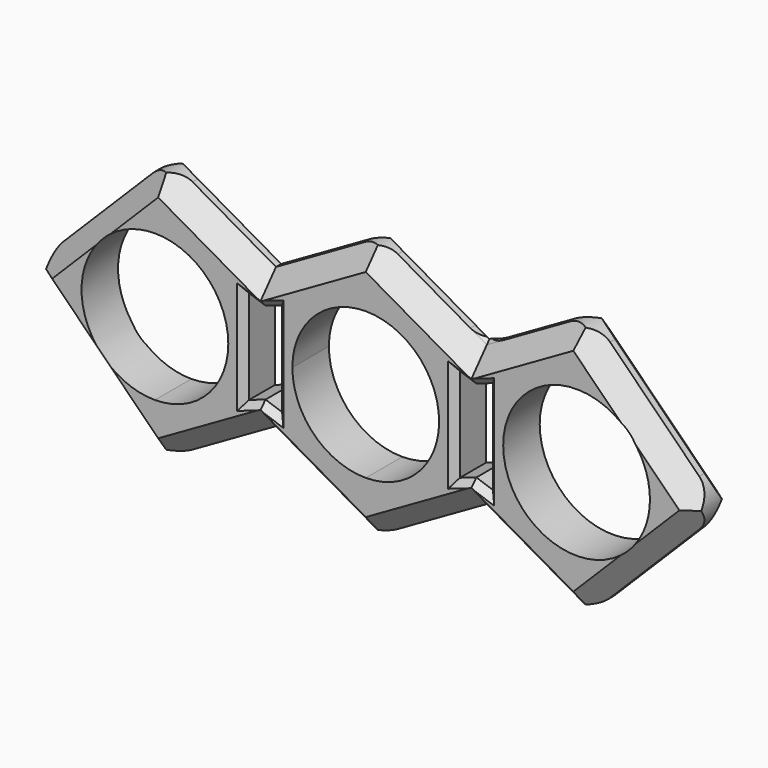
from build123d import *

# Parameters (mm, degrees)
F1_DEPTH      = 7
F3_DEPTH      = 127
F4_T1_DEPTH   = 43.7143691753
F4_T3_DEPTH   = 43.7143691753
F4_T5_DEPTH   = 43.7143691753
F4_T7_DEPTH   = 43.7143691753
F4_T12_DEPTH  = 34.0552517656
F4_T17_DEPTH  = 34.0552517656
F4_T22_DEPTH  = 34.0552517656
F4_T27_DEPTH  = 34.0552517656
F4_T32_DEPTH  = 34.0552517656
F4_T37_DEPTH  = 34.0552517656
F4_T42_DEPTH  = 34.0552517656
F4_T47_DEPTH  = 34.0552517656
F4_T52_DEPTH  = 34.0552517656
F4_T57_DEPTH  = 34.0552517656
F4_T62_DEPTH  = 34.0552517656
F4_T67_DEPTH  = 34.0552517656
F4_T72_DEPTH  = 34.0552517656
F4_T77_DEPTH  = 34.0552517656
F4_T82_DEPTH  = 34.0552517656
F4_T87_DEPTH  = 34.0552517656
F4_T93_DEPTH  = 34.0552517656
F4_T97_DEPTH  = 34.0552517656
F4_T104_DEPTH = 34.0552517656
F4_T108_DEPTH = 34.0552517656
F4_T115_DEPTH = 34.0552517656
F4_T119_DEPTH = 34.0552517656
F4_T126_DEPTH = 34.0552517656
F4_T130_DEPTH = 34.0552517656
F4_T137_DEPTH = 34.0552517656
F4_T141_DEPTH = 34.0552517656
F4_T148_DEPTH = 34.0552517656
F4_T152_DEPTH = 34.0552517656
F4_T159_DEPTH = 34.0552517656
F4_T163_DEPTH = 34.0552517656
F4_T170_DEPTH = 34.0552517656
F4_T174_DEPTH = 34.0552517656
F5_T4_DEPTH   = 15.5437371567
F5_T10_DEPTH  = 15.5437371567
F5_T16_DEPTH  = 15.5437371567
F5_T19_DEPTH  = 26.4
F5_T21_DEPTH  = 20.4179884798
F5_T23_DEPTH  = 15.5437371567
F6_T4_DEPTH   = 19.5677673114
F6_T10_DEPTH  = 19.5677673114
F6_T16_DEPTH  = 19.5677673114
F6_T22_DEPTH  = 19.5677673114
F6_T28_DEPTH  = 19.5677673114
F6_T34_DEPTH  = 19.5677673114
F6_T40_DEPTH  = 19.5677673114
F6_T46_DEPTH  = 19.5677673114
F6_T52_DEPTH  = 7.8272082618
F6_T57_DEPTH  = 7.8272082618
F6_T62_DEPTH  = 7.8272082618
F6_T67_DEPTH  = 7.8272082618
F6_T72_DEPTH  = 7.8272082618
F6_T77_DEPTH  = 7.8272082618
F6_T82_DEPTH  = 7.8272082618
F6_T87_DEPTH  = 7.8272082618
F6_T92_DEPTH  = 7.8272082618
F6_T97_DEPTH  = 7.8272082618
F6_T102_DEPTH = 7.8272082618
F6_T107_DEPTH = 7.8272082618
F6_T112_DEPTH = 7.8272082618
F6_T117_DEPTH = 7.8272082618
F6_T122_DEPTH = 7.8272082618
F6_T127_DEPTH = 7.8272082618
F6_T133_DEPTH = 7.8272082618
F6_T137_DEPTH = 19.5677673114
F6_T144_DEPTH = 7.8272082618
F6_T148_DEPTH = 19.5677673114
F6_T155_DEPTH = 19.5677673114
F6_T159_DEPTH = 7.8272082618
F6_T166_DEPTH = 7.8272082618
F6_T170_DEPTH = 19.5677673114
F6_T177_DEPTH = 19.5677673114
F6_T181_DEPTH = 7.8272082618
F6_T188_DEPTH = 7.8272082618
F6_T192_DEPTH = 19.5677673114
F6_T199_DEPTH = 7.8272082618
F6_T203_DEPTH = 19.5677673114
F6_T210_DEPTH = 7.8272082618
F6_T214_DEPTH = 19.5677673114
F6_T221_DEPTH = 7.8272082618
F6_T225_DEPTH = 19.5677673114
F6_T232_DEPTH = 7.8272082618
F6_T236_DEPTH = 19.5677673114
F6_T243_DEPTH = 19.5677673114
F6_T247_DEPTH = 7.8272082618
F6_T254_DEPTH = 7.8272082618
F6_T258_DEPTH = 19.5677673114
F6_T265_DEPTH = 19.5677673114
F6_T269_DEPTH = 7.8272082618
F6_T276_DEPTH = 7.8272082618
F6_T280_DEPTH = 19.5677673114
F6_T287_DEPTH = 7.8272082618
F6_T291_DEPTH = 19.5677673114
F6_T298_DEPTH = 7.8272082618
F6_T302_DEPTH = 19.5677673114


# Not quite as in the source:
# - a fillet or chamfer that OpenCascade refuses, or shapes differently, is made with other operations: its cross-section is extruded or revolved along the edge and cut away or added


with BuildPart() as f1:
    # F0 (on Front) → F1 (new body)
    with BuildSketch(Plane.XZ):
        with BuildLine():
            Line((16.1630827934, 10.7452115044), (16.1630827934, 0))
            Line((16.1630827934, 0), (21.0761655867, 0))
            ThreePointArc((21.0761655867, 0), (32.3261655867, 11.25), (43.5761655867, 0))
            Line((43.5761655867, 0), (52.3261655867, 0))
            Line((52.3261655867, 0), (32.3261655867, 20))
            Line((32.3261655867, 20), (16.1630827934, 10.7452115044))
        make_face()
        with BuildLine():
            Line((21.0761655867, 0), (16.1630827934, 0))
            Line((16.1630827934, 0), (16.1630827934, -10.7452115044))
            Line((16.1630827934, -10.7452115044), (32.3261655867, -20))
            Line((32.3261655867, -20), (52.3261655867, 0))
            Line((52.3261655867, 0), (43.5761655867, 0))
            ThreePointArc((43.5761655867, 0), (32.3261655867, -11.25), (21.0761655867, 0))
        make_face()
        with BuildLine():
            Line((16.1630827934, 0), (11.25, 0))
            ThreePointArc((11.25, 0), (7.9549512883, -7.9549512883), (0, -11.25))
            Line((0, -11.25), (0, -20))
            Line((0, -20), (16.1630827934, -10.7452115044))
            Line((16.1630827934, -10.7452115044), (16.1630827934, 0))
        make_face()
        with BuildLine():
            ThreePointArc((0, 11.25), (7.9549512883, 7.9549512883), (11.25, 0))
            Line((11.25, 0), (16.1630827934, 0))
            Line((16.1630827934, 0), (16.1630827934, 10.7452115044))
            Line((16.1630827934, 10.7452115044), (0, 20))
            Line((0, 20), (0, 11.25))
        make_face()
        with BuildLine():
            ThreePointArc((-11.25, 0), (-7.9549512883, 7.9549512883), (0, 11.25))
            Line((0, 11.25), (0, 20))
            Line((0, 20), (-16.1630827934, 10.7452115044))
            Line((-16.1630827934, 10.7452115044), (-16.1630827934, 0))
            Line((-16.1630827934, 0), (-11.25, 0))
        make_face()
        with BuildLine():
            Line((0, -20), (0, -11.25))
            ThreePointArc((0, -11.25), (-7.9549512883, -7.9549512883), (-11.25, 0))
            Line((-11.25, 0), (-16.1630827934, 0))
            Line((-16.1630827934, 0), (-16.1630827934, -10.7452115044))
            Line((-16.1630827934, -10.7452115044), (0, -20))
        make_face()
        with BuildLine():
            Line((-16.1630827934, -10.7452115044), (-16.1630827934, 0))
            Line((-16.1630827934, 0), (-21.0761655867, 0))
            ThreePointArc((-21.0761655867, 0), (-24.3712142984, -7.9549512883), (-32.3261655867, -11.25))
            Line((-32.3261655867, -11.25), (-32.3261655867, -20))
            Line((-32.3261655867, -20), (-16.1630827934, -10.7452115044))
        make_face()
        with BuildLine():
            Line((-52.3261655867, 0), (-32.3261655867, -20))
            Line((-32.3261655867, -20), (-32.3261655867, -11.25))
            ThreePointArc((-32.3261655867, -11.25), (-40.2811168751, -7.9549512883), (-43.5761655867, 0))
            Line((-43.5761655867, 0), (-52.3261655867, 0))
        make_face()
        with BuildLine():
            Line((-32.3261655867, 11.25), (-32.3261655867, 20))
            Line((-32.3261655867, 20), (-52.3261655867, 0))
            Line((-52.3261655867, 0), (-43.5761655867, 0))
            ThreePointArc((-43.5761655867, 0), (-40.2811168751, 7.9549512883), (-32.3261655867, 11.25))
        make_face()
        with BuildLine():
            Line((-21.0761655867, 0), (-16.1630827934, 0))
            Line((-16.1630827934, 0), (-16.1630827934, 10.7452115044))
            Line((-16.1630827934, 10.7452115044), (-32.3261655867, 20))
            Line((-32.3261655867, 20), (-32.3261655867, 11.25))
            ThreePointArc((-32.3261655867, 11.25), (-24.3712142984, 7.9549512883), (-21.0761655867, 0))
        make_face()
    extrude(amount=F1_DEPTH)

    # F2 (on face) → F3 (cut)
    with BuildSketch(Plane.XZ.offset(7)):
        Polygon((-16.1630827934, 6.3396666324), (-16.1630827934, -6.3396666324), (-13.6250335872, -7.2122006677), (-13.6250335872, 7.2122006677), align=None)
        Polygon((-18.7011319995, -7.2122006677), (-16.1630827934, -6.3396666324), (-16.1630827934, 6.3396666324), (-18.7011319995, 7.2122006677), align=None)
        Polygon((13.6250335872, -7.2122006677), (16.1630827934, -6.3396666324), (16.1630827934, 6.3396666324), (13.6250335872, 7.2122006677), align=None)
        Polygon((16.1630827934, 6.3396666324), (16.1630827934, -6.3396666324), (18.7011319995, -7.2122006677), (18.7011319995, 7.2122006677), align=None)
    extrude(amount=-F3_DEPTH, mode=Mode.SUBTRACT)

    # F4: chamfer of 3 on 24 edges, made by hand

    # F4_s2 → F4_t1 (cut)
    with BuildSketch(Plane(origin=(31.6184462329, 0, -31.6184462329), x_dir=(0, 1, 0), z_dir=(-0.7071067812, 0, 0.7071067812))):
        Polygon((-7, -34.0001865199), (-4, -37.0001865199), (-7, -37.0001865199), align=None)
        Polygon((0, -34.0001865199), (-3, -37.0001865199), (0, -37.0001865199), align=None)
    extrude(amount=F4_T1_DEPTH, mode=Mode.SUBTRACT)

    # F4_s4 → F4_t3 (cut)
    with BuildSketch(Plane(origin=(-0.7077193538, 0, -0.7077193538), x_dir=(0, 1, 0), z_dir=(-0.7071067812, 0, -0.7071067812))):
        Polygon((-7, -34.0001865199), (-4, -37.0001865199), (-7, -37.0001865199), align=None)
        Polygon((0, -34.0001865199), (-3, -37.0001865199), (0, -37.0001865199), align=None)
    extrude(amount=F4_T3_DEPTH, mode=Mode.SUBTRACT)

    # F4_s6 → F4_t5 (cut)
    with BuildSketch(Plane(origin=(-31.6184462329, 0, 31.6184462329), x_dir=(0, 1, 0), z_dir=(0.7071067812, 0, -0.7071067812))):
        Polygon((-7, -34.0001865199), (-4, -37.0001865199), (-7, -37.0001865199), align=None)
        Polygon((0, -34.0001865199), (-3, -37.0001865199), (0, -37.0001865199), align=None)
    extrude(amount=F4_T5_DEPTH, mode=Mode.SUBTRACT)

    # F4_s8 → F4_t7 (cut)
    with BuildSketch(Plane(origin=(0.7077193538, 0, 0.7077193538), x_dir=(0, 1, 0), z_dir=(0.7071067812, 0, 0.7071067812))):
        Polygon((0, -34.0001865199), (-3, -37.0001865199), (0, -37.0001865199), align=None)
        Polygon((-7, -34.0001865199), (-4, -37.0001865199), (-7, -37.0001865199), align=None)
    extrude(amount=F4_T7_DEPTH, mode=Mode.SUBTRACT)


with BuildPart() as f4_tool10:
    # F4_s11 → F4_t12 (new body)
    with BuildSketch(Plane(origin=(-10.1105795702, 0, 5.7891973138), x_dir=(0, 1, 0), z_dir=(-0.8678093579, 0, 0.4968972915))):
        Polygon((-7, 1.7065969657), (-4, -1.2934030343), (-7, -1.2934030343), align=None)
    extrude(amount=F4_T12_DEPTH)

    split(bisect_by=Plane(origin=(-8.6242423897, 0, 15.0618616342), x_dir=(0, 1, 0), z_dir=(-0.4968972915, 0, 0.8678093579)), keep=Keep.TOP)


with BuildPart() as f1_1:
    add(f1.part)

    # F4_t9: cut F4_tool10
    add(f4_tool10.part, mode=Mode.SUBTRACT)


with BuildPart() as f4_tool15:
    # F4_s16 → F4_t17 (new body)
    with BuildSketch(Plane(origin=(15.3194340774, 0, 8.7717252997), x_dir=(0, 1, 0), z_dir=(-0.8678093579, 0, -0.4968972915))):
        Polygon((-7, -14.3561871586), (-4, -17.3561871586), (-7, -17.3561871586), align=None)
    extrude(amount=F4_T17_DEPTH)

    split(bisect_by=Plane(origin=(0.6426884646, 0, 1.1224272567), x_dir=(0, 1, 0), z_dir=(0.4968972915, 0, 0.8678093579)), keep=Keep.TOP)


with BuildPart() as f1_2:
    add(f1_1.part)

    # F4_t14: cut F4_tool15
    add(f4_tool15.part, mode=Mode.SUBTRACT)


with BuildPart() as f4_tool20:
    # F4_s21 → F4_t22 (new body)
    with BuildSketch(Plane(origin=(14.2340320914, 0, -8.1502370637), x_dir=(0, 1, 0), z_dir=(-0.8678093579, 0, 0.4968972915))):
        Polygon((-7, -14.3561871586), (-4, -17.3561871586), (-7, -17.3561871586), align=None)
    extrude(amount=F4_T22_DEPTH)

    split(bisect_by=Plane(origin=(-0.6426884646, 0, 1.1224272567), x_dir=(0, 1, 0), z_dir=(-0.4968972915, 0, 0.8678093579)), keep=Keep.TOP)


with BuildPart() as f1_3:
    add(f1_2.part)

    # F4_t19: cut F4_tool20
    add(f4_tool20.part, mode=Mode.SUBTRACT)


with BuildPart() as f4_tool25:
    # F4_s26 → F4_t27 (new body)
    with BuildSketch(Plane(origin=(39.664045739, 0, 22.7111596771), x_dir=(0, 1, 0), z_dir=(-0.8678093579, 0, -0.4968972915))):
        Polygon((-7, 1.7065969657), (-4, -1.2934030343), (-7, -1.2934030343), align=None)
    extrude(amount=F4_T27_DEPTH)

    split(bisect_by=Plane(origin=(8.6242423897, 0, 15.0618616342), x_dir=(0, 1, 0), z_dir=(0.4968972915, 0, 0.8678093579)), keep=Keep.TOP)


with BuildPart() as f1_4:
    add(f1_3.part)

    # F4_t24: cut F4_tool25
    add(f4_tool25.part, mode=Mode.SUBTRACT)


with BuildPart() as f4_tool30:
    # F4_s31 → F4_t32 (new body)
    with BuildSketch(Plane(origin=(39.664045739, 0, 22.7111596771), x_dir=(0, 1, 0), z_dir=(-0.8678093579, 0, -0.4968972915))):
        Polygon((0, 1.7065969657), (-3, -1.2934030343), (0, -1.2934030343), align=None)
    extrude(amount=F4_T32_DEPTH)

    split(bisect_by=Plane(origin=(8.6242423897, 0, 15.0618616342), x_dir=(0, 1, 0), z_dir=(0.4968972915, 0, 0.8678093579)), keep=Keep.TOP)


with BuildPart() as f1_5:
    add(f1_4.part)

    # F4_t29: cut F4_tool30
    add(f4_tool30.part, mode=Mode.SUBTRACT)


with BuildPart() as f4_tool35:
    # F4_s36 → F4_t37 (new body)
    with BuildSketch(Plane(origin=(14.2340320914, 0, -8.1502370637), x_dir=(0, 1, 0), z_dir=(-0.8678093579, 0, 0.4968972915))):
        Polygon((0, -14.3561871586), (-3, -17.3561871586), (0, -17.3561871586), align=None)
    extrude(amount=F4_T37_DEPTH)

    split(bisect_by=Plane(origin=(-0.6426884646, 0, 1.1224272567), x_dir=(0, 1, 0), z_dir=(-0.4968972915, 0, 0.8678093579)), keep=Keep.TOP)


with BuildPart() as f1_6:
    add(f1_5.part)

    # F4_t34: cut F4_tool35
    add(f4_tool35.part, mode=Mode.SUBTRACT)


with BuildPart() as f4_tool40:
    # F4_s41 → F4_t42 (new body)
    with BuildSketch(Plane(origin=(15.3194340774, 0, 8.7717252997), x_dir=(0, 1, 0), z_dir=(-0.8678093579, 0, -0.4968972915))):
        Polygon((0, -14.3561871586), (-3, -17.3561871586), (0, -17.3561871586), align=None)
    extrude(amount=F4_T42_DEPTH)

    split(bisect_by=Plane(origin=(0.6426884646, 0, 1.1224272567), x_dir=(0, 1, 0), z_dir=(0.4968972915, 0, 0.8678093579)), keep=Keep.TOP)


with BuildPart() as f1_7:
    add(f1_6.part)

    # F4_t39: cut F4_tool40
    add(f4_tool40.part, mode=Mode.SUBTRACT)


with BuildPart() as f4_tool45:
    # F4_s46 → F4_t47 (new body)
    with BuildSketch(Plane(origin=(-10.1105795702, 0, 5.7891973138), x_dir=(0, 1, 0), z_dir=(-0.8678093579, 0, 0.4968972915))):
        Polygon((0, 1.7065969657), (-3, -1.2934030343), (0, -1.2934030343), align=None)
    extrude(amount=F4_T47_DEPTH)

    split(bisect_by=Plane(origin=(-8.6242423897, 0, 15.0618616342), x_dir=(0, 1, 0), z_dir=(-0.4968972915, 0, 0.8678093579)), keep=Keep.TOP)


with BuildPart() as f1_8:
    add(f1_7.part)

    # F4_t44: cut F4_tool45
    add(f4_tool45.part, mode=Mode.SUBTRACT)


with BuildPart() as f4_tool50:
    # F4_s51 → F4_t52 (new body)
    with BuildSketch(Plane(origin=(-39.664045739, 0, -22.7111596771), x_dir=(0, 1, 0), z_dir=(0.8678093579, 0, 0.4968972915))):
        Polygon((0, 1.7065969657), (-3, -1.2934030343), (0, -1.2934030343), align=None)
    extrude(amount=F4_T52_DEPTH)

    split(bisect_by=Plane(origin=(-8.6242423897, 0, -15.0618616342), x_dir=(0, 1, 0), z_dir=(-0.4968972915, 0, -0.8678093579)), keep=Keep.TOP)


with BuildPart() as f1_9:
    add(f1_8.part)

    # F4_t49: cut F4_tool50
    add(f4_tool50.part, mode=Mode.SUBTRACT)


with BuildPart() as f4_tool55:
    # F4_s56 → F4_t57 (new body)
    with BuildSketch(Plane(origin=(-39.664045739, 0, -22.7111596771), x_dir=(0, 1, 0), z_dir=(0.8678093579, 0, 0.4968972915))):
        Polygon((-7, 1.7065969657), (-4, -1.2934030343), (-7, -1.2934030343), align=None)
    extrude(amount=F4_T57_DEPTH)

    split(bisect_by=Plane(origin=(-8.6242423897, 0, -15.0618616342), x_dir=(0, 1, 0), z_dir=(-0.4968972915, 0, -0.8678093579)), keep=Keep.TOP)


with BuildPart() as f1_10:
    add(f1_9.part)

    # F4_t54: cut F4_tool55
    add(f4_tool55.part, mode=Mode.SUBTRACT)


with BuildPart() as f4_tool60:
    # F4_s61 → F4_t62 (new body)
    with BuildSketch(Plane(origin=(-14.2340320914, 0, 8.1502370637), x_dir=(0, 1, 0), z_dir=(0.8678093579, 0, -0.4968972915))):
        Polygon((-4, -17.3561871586), (-7, -14.3561871586), (-7, -17.3561871586), align=None)
    extrude(amount=F4_T62_DEPTH)

    split(bisect_by=Plane(origin=(0.6426884646, 0, -1.1224272567), x_dir=(0, 1, 0), z_dir=(0.4968972915, 0, -0.8678093579)), keep=Keep.TOP)


with BuildPart() as f1_11:
    add(f1_10.part)

    # F4_t59: cut F4_tool60
    add(f4_tool60.part, mode=Mode.SUBTRACT)


with BuildPart() as f4_tool65:
    # F4_s66 → F4_t67 (new body)
    with BuildSketch(Plane(origin=(-14.2340320914, 0, 8.1502370637), x_dir=(0, 1, 0), z_dir=(0.8678093579, 0, -0.4968972915))):
        Polygon((-3, -17.3561871586), (0, -14.3561871586), (0, -17.3561871586), align=None)
    extrude(amount=F4_T67_DEPTH)

    split(bisect_by=Plane(origin=(0.6426884646, 0, -1.1224272567), x_dir=(0, 1, 0), z_dir=(0.4968972915, 0, -0.8678093579)), keep=Keep.TOP)


with BuildPart() as f1_12:
    add(f1_11.part)

    # F4_t64: cut F4_tool65
    add(f4_tool65.part, mode=Mode.SUBTRACT)


with BuildPart() as f4_tool70:
    # F4_s71 → F4_t72 (new body)
    with BuildSketch(Plane(origin=(-15.3194340774, 0, -8.7717252997), x_dir=(0, 1, 0), z_dir=(0.8678093579, 0, 0.4968972915))):
        Polygon((-3, -17.3561871586), (0, -14.3561871586), (0, -17.3561871586), align=None)
    extrude(amount=F4_T72_DEPTH)

    split(bisect_by=Plane(origin=(-0.6426884646, 0, -1.1224272567), x_dir=(0, 1, 0), z_dir=(-0.4968972915, 0, -0.8678093579)), keep=Keep.TOP)


with BuildPart() as f1_13:
    add(f1_12.part)

    # F4_t69: cut F4_tool70
    add(f4_tool70.part, mode=Mode.SUBTRACT)


with BuildPart() as f4_tool75:
    # F4_s76 → F4_t77 (new body)
    with BuildSketch(Plane(origin=(-15.3194340774, 0, -8.7717252997), x_dir=(0, 1, 0), z_dir=(0.8678093579, 0, 0.4968972915))):
        Polygon((-4, -17.3561871586), (-7, -14.3561871586), (-7, -17.3561871586), align=None)
    extrude(amount=F4_T77_DEPTH)

    split(bisect_by=Plane(origin=(-0.6426884646, 0, -1.1224272567), x_dir=(0, 1, 0), z_dir=(-0.4968972915, 0, -0.8678093579)), keep=Keep.TOP)


with BuildPart() as f1_14:
    add(f1_13.part)

    # F4_t74: cut F4_tool75
    add(f4_tool75.part, mode=Mode.SUBTRACT)


with BuildPart() as f4_tool80:
    # F4_s81 → F4_t82 (new body)
    with BuildSketch(Plane(origin=(10.1105795702, 0, -5.7891973138), x_dir=(0, 1, 0), z_dir=(0.8678093579, 0, -0.4968972915))):
        Polygon((-3, -1.2934030343), (0, 1.7065969657), (0, -1.2934030343), align=None)
    extrude(amount=F4_T82_DEPTH)

    split(bisect_by=Plane(origin=(8.6242423897, 0, -15.0618616342), x_dir=(0, 1, 0), z_dir=(0.4968972915, 0, -0.8678093579)), keep=Keep.TOP)


with BuildPart() as f1_15:
    add(f1_14.part)

    # F4_t79: cut F4_tool80
    add(f4_tool80.part, mode=Mode.SUBTRACT)


with BuildPart() as f4_tool85:
    # F4_s86 → F4_t87 (new body)
    with BuildSketch(Plane(origin=(10.1105795702, 0, -5.7891973138), x_dir=(0, 1, 0), z_dir=(0.8678093579, 0, -0.4968972915))):
        Polygon((-4, -1.2934030343), (-7, 1.7065969657), (-7, -1.2934030343), align=None)
    extrude(amount=F4_T87_DEPTH)

    split(bisect_by=Plane(origin=(8.6242423897, 0, -15.0618616342), x_dir=(0, 1, 0), z_dir=(0.4968972915, 0, -0.8678093579)), keep=Keep.TOP)


with BuildPart() as f1_16:
    add(f1_15.part)

    # F4_t84: cut F4_tool85
    add(f4_tool85.part, mode=Mode.SUBTRACT)


with BuildPart() as f4_tool91:
    # F4_s92 → F4_t93 (new body)
    with BuildSketch(Plane(origin=(-10.1105795702, 0, 5.7891973138), x_dir=(0, 1, 0), z_dir=(-0.8678093579, 0, 0.4968972915))):
        Polygon((-7, 1.7065969657), (-4, -1.2934030343), (-7, -1.2934030343), align=None)
    extrude(amount=F4_T93_DEPTH)

    split(bisect_by=Plane(origin=(-8.6242423897, 0, 15.0618616342), x_dir=(0, 1, 0), z_dir=(0.4968972915, 0, -0.8678093579)), keep=Keep.TOP)


with BuildPart() as f4_tool95:
    # F4_s96 → F4_t97 (new body)
    with BuildSketch(Plane(origin=(15.3194340774, 0, 8.7717252997), x_dir=(0, 1, 0), z_dir=(-0.8678093579, 0, -0.4968972915))):
        Polygon((-7, -14.3561871586), (-4, -17.3561871586), (-7, -17.3561871586), align=None)
    extrude(amount=F4_T97_DEPTH)

    split(bisect_by=Plane(origin=(0.6426884646, 0, 1.1224272567), x_dir=(0, 1, 0), z_dir=(-0.4968972915, 0, -0.8678093579)), keep=Keep.TOP)


with BuildPart() as f4_tool91_1:
    add(f4_tool91.part)

    # F4_t99: intersect F4_tool95
    add(f4_tool95.part, mode=Mode.INTERSECT)


with BuildPart() as f1_17:
    add(f1_16.part)

    # F4_t89: cut F4_tool91
    add(f4_tool91_1.part, mode=Mode.SUBTRACT)


with BuildPart() as f4_tool102:
    # F4_s103 → F4_t104 (new body)
    with BuildSketch(Plane(origin=(39.664045739, 0, 22.7111596771), x_dir=(0, 1, 0), z_dir=(-0.8678093579, 0, -0.4968972915))):
        Polygon((-7, 1.7065969657), (-4, -1.2934030343), (-7, -1.2934030343), align=None)
    extrude(amount=F4_T104_DEPTH)

    split(bisect_by=Plane(origin=(8.6242423897, 0, 15.0618616342), x_dir=(0, 1, 0), z_dir=(-0.4968972915, 0, -0.8678093579)), keep=Keep.TOP)


with BuildPart() as f4_tool106:
    # F4_s107 → F4_t108 (new body)
    with BuildSketch(Plane(origin=(14.2340320914, 0, -8.1502370637), x_dir=(0, 1, 0), z_dir=(-0.8678093579, 0, 0.4968972915))):
        Polygon((-7, -14.3561871586), (-4, -17.3561871586), (-7, -17.3561871586), align=None)
    extrude(amount=F4_T108_DEPTH)

    split(bisect_by=Plane(origin=(-0.6426884646, 0, 1.1224272567), x_dir=(0, 1, 0), z_dir=(0.4968972915, 0, -0.8678093579)), keep=Keep.TOP)


with BuildPart() as f4_tool102_1:
    add(f4_tool102.part)

    # F4_t110: intersect F4_tool106
    add(f4_tool106.part, mode=Mode.INTERSECT)


with BuildPart() as f1_18:
    add(f1_17.part)

    # F4_t100: cut F4_tool102
    add(f4_tool102_1.part, mode=Mode.SUBTRACT)


with BuildPart() as f4_tool113:
    # F4_s114 → F4_t115 (new body)
    with BuildSketch(Plane(origin=(39.664045739, 0, 22.7111596771), x_dir=(0, 1, 0), z_dir=(-0.8678093579, 0, -0.4968972915))):
        Polygon((0, 1.7065969657), (-3, -1.2934030343), (0, -1.2934030343), align=None)
    extrude(amount=F4_T115_DEPTH)

    split(bisect_by=Plane(origin=(8.6242423897, 0, 15.0618616342), x_dir=(0, 1, 0), z_dir=(-0.4968972915, 0, -0.8678093579)), keep=Keep.TOP)


with BuildPart() as f4_tool117:
    # F4_s118 → F4_t119 (new body)
    with BuildSketch(Plane(origin=(14.2340320914, 0, -8.1502370637), x_dir=(0, 1, 0), z_dir=(-0.8678093579, 0, 0.4968972915))):
        Polygon((0, -14.3561871586), (-3, -17.3561871586), (0, -17.3561871586), align=None)
    extrude(amount=F4_T119_DEPTH)

    split(bisect_by=Plane(origin=(-0.6426884646, 0, 1.1224272567), x_dir=(0, 1, 0), z_dir=(0.4968972915, 0, -0.8678093579)), keep=Keep.TOP)


with BuildPart() as f4_tool113_1:
    add(f4_tool113.part)

    # F4_t121: intersect F4_tool117
    add(f4_tool117.part, mode=Mode.INTERSECT)


with BuildPart() as f1_19:
    add(f1_18.part)

    # F4_t111: cut F4_tool113
    add(f4_tool113_1.part, mode=Mode.SUBTRACT)


with BuildPart() as f4_tool124:
    # F4_s125 → F4_t126 (new body)
    with BuildSketch(Plane(origin=(-10.1105795702, 0, 5.7891973138), x_dir=(0, 1, 0), z_dir=(-0.8678093579, 0, 0.4968972915))):
        Polygon((0, 1.7065969657), (-3, -1.2934030343), (0, -1.2934030343), align=None)
    extrude(amount=F4_T126_DEPTH)

    split(bisect_by=Plane(origin=(-8.6242423897, 0, 15.0618616342), x_dir=(0, 1, 0), z_dir=(0.4968972915, 0, -0.8678093579)), keep=Keep.TOP)


with BuildPart() as f4_tool128:
    # F4_s129 → F4_t130 (new body)
    with BuildSketch(Plane(origin=(15.3194340774, 0, 8.7717252997), x_dir=(0, 1, 0), z_dir=(-0.8678093579, 0, -0.4968972915))):
        Polygon((0, -14.3561871586), (-3, -17.3561871586), (0, -17.3561871586), align=None)
    extrude(amount=F4_T130_DEPTH)

    split(bisect_by=Plane(origin=(0.6426884646, 0, 1.1224272567), x_dir=(0, 1, 0), z_dir=(-0.4968972915, 0, -0.8678093579)), keep=Keep.TOP)


with BuildPart() as f4_tool124_1:
    add(f4_tool124.part)

    # F4_t132: intersect F4_tool128
    add(f4_tool128.part, mode=Mode.INTERSECT)


with BuildPart() as f1_20:
    add(f1_19.part)

    # F4_t122: cut F4_tool124
    add(f4_tool124_1.part, mode=Mode.SUBTRACT)


with BuildPart() as f4_tool135:
    # F4_s136 → F4_t137 (new body)
    with BuildSketch(Plane(origin=(-14.2340320914, 0, 8.1502370637), x_dir=(0, 1, 0), z_dir=(0.8678093579, 0, -0.4968972915))):
        Polygon((-3, -17.3561871586), (0, -14.3561871586), (0, -17.3561871586), align=None)
    extrude(amount=F4_T137_DEPTH)

    split(bisect_by=Plane(origin=(0.6426884646, 0, -1.1224272567), x_dir=(0, 1, 0), z_dir=(-0.4968972915, 0, 0.8678093579)), keep=Keep.TOP)


with BuildPart() as f4_tool139:
    # F4_s140 → F4_t141 (new body)
    with BuildSketch(Plane(origin=(-39.664045739, 0, -22.7111596771), x_dir=(0, 1, 0), z_dir=(0.8678093579, 0, 0.4968972915))):
        Polygon((0, 1.7065969657), (-3, -1.2934030343), (0, -1.2934030343), align=None)
    extrude(amount=F4_T141_DEPTH)

    split(bisect_by=Plane(origin=(-8.6242423897, 0, -15.0618616342), x_dir=(0, 1, 0), z_dir=(0.4968972915, 0, 0.8678093579)), keep=Keep.TOP)


with BuildPart() as f4_tool135_1:
    add(f4_tool135.part)

    # F4_t143: intersect F4_tool139
    add(f4_tool139.part, mode=Mode.INTERSECT)


with BuildPart() as f1_21:
    add(f1_20.part)

    # F4_t133: cut F4_tool135
    add(f4_tool135_1.part, mode=Mode.SUBTRACT)


with BuildPart() as f4_tool146:
    # F4_s147 → F4_t148 (new body)
    with BuildSketch(Plane(origin=(-14.2340320914, 0, 8.1502370637), x_dir=(0, 1, 0), z_dir=(0.8678093579, 0, -0.4968972915))):
        Polygon((-4, -17.3561871586), (-7, -14.3561871586), (-7, -17.3561871586), align=None)
    extrude(amount=F4_T148_DEPTH)

    split(bisect_by=Plane(origin=(0.6426884646, 0, -1.1224272567), x_dir=(0, 1, 0), z_dir=(-0.4968972915, 0, 0.8678093579)), keep=Keep.TOP)


with BuildPart() as f4_tool150:
    # F4_s151 → F4_t152 (new body)
    with BuildSketch(Plane(origin=(-39.664045739, 0, -22.7111596771), x_dir=(0, 1, 0), z_dir=(0.8678093579, 0, 0.4968972915))):
        Polygon((-7, 1.7065969657), (-4, -1.2934030343), (-7, -1.2934030343), align=None)
    extrude(amount=F4_T152_DEPTH)

    split(bisect_by=Plane(origin=(-8.6242423897, 0, -15.0618616342), x_dir=(0, 1, 0), z_dir=(0.4968972915, 0, 0.8678093579)), keep=Keep.TOP)


with BuildPart() as f4_tool146_1:
    add(f4_tool146.part)

    # F4_t154: intersect F4_tool150
    add(f4_tool150.part, mode=Mode.INTERSECT)


with BuildPart() as f1_22:
    add(f1_21.part)

    # F4_t144: cut F4_tool146
    add(f4_tool146_1.part, mode=Mode.SUBTRACT)


with BuildPart() as f4_tool157:
    # F4_s158 → F4_t159 (new body)
    with BuildSketch(Plane(origin=(-15.3194340774, 0, -8.7717252997), x_dir=(0, 1, 0), z_dir=(0.8678093579, 0, 0.4968972915))):
        Polygon((-3, -17.3561871586), (0, -14.3561871586), (0, -17.3561871586), align=None)
    extrude(amount=F4_T159_DEPTH)

    split(bisect_by=Plane(origin=(-0.6426884646, 0, -1.1224272567), x_dir=(0, 1, 0), z_dir=(0.4968972915, 0, 0.8678093579)), keep=Keep.TOP)


with BuildPart() as f4_tool161:
    # F4_s162 → F4_t163 (new body)
    with BuildSketch(Plane(origin=(10.1105795702, 0, -5.7891973138), x_dir=(0, 1, 0), z_dir=(0.8678093579, 0, -0.4968972915))):
        Polygon((-3, -1.2934030343), (0, 1.7065969657), (0, -1.2934030343), align=None)
    extrude(amount=F4_T163_DEPTH)

    split(bisect_by=Plane(origin=(8.6242423897, 0, -15.0618616342), x_dir=(0, 1, 0), z_dir=(-0.4968972915, 0, 0.8678093579)), keep=Keep.TOP)


with BuildPart() as f4_tool157_1:
    add(f4_tool157.part)

    # F4_t165: intersect F4_tool161
    add(f4_tool161.part, mode=Mode.INTERSECT)


with BuildPart() as f1_23:
    add(f1_22.part)

    # F4_t155: cut F4_tool157
    add(f4_tool157_1.part, mode=Mode.SUBTRACT)


with BuildPart() as f4_tool168:
    # F4_s169 → F4_t170 (new body)
    with BuildSketch(Plane(origin=(-15.3194340774, 0, -8.7717252997), x_dir=(0, 1, 0), z_dir=(0.8678093579, 0, 0.4968972915))):
        Polygon((-4, -17.3561871586), (-7, -14.3561871586), (-7, -17.3561871586), align=None)
    extrude(amount=F4_T170_DEPTH)

    split(bisect_by=Plane(origin=(-0.6426884646, 0, -1.1224272567), x_dir=(0, 1, 0), z_dir=(0.4968972915, 0, 0.8678093579)), keep=Keep.TOP)


with BuildPart() as f4_tool172:
    # F4_s173 → F4_t174 (new body)
    with BuildSketch(Plane(origin=(10.1105795702, 0, -5.7891973138), x_dir=(0, 1, 0), z_dir=(0.8678093579, 0, -0.4968972915))):
        Polygon((-4, -1.2934030343), (-7, 1.7065969657), (-7, -1.2934030343), align=None)
    extrude(amount=F4_T174_DEPTH)

    split(bisect_by=Plane(origin=(8.6242423897, 0, -15.0618616342), x_dir=(0, 1, 0), z_dir=(-0.4968972915, 0, 0.8678093579)), keep=Keep.TOP)


with BuildPart() as f4_tool168_1:
    add(f4_tool168.part)

    # F4_t176: intersect F4_tool172
    add(f4_tool172.part, mode=Mode.INTERSECT)


with BuildPart() as f1_24:
    add(f1_23.part)

    # F4_t166: cut F4_tool168
    add(f4_tool168_1.part, mode=Mode.SUBTRACT)

    # F5: fillet of radius 5.08 on 9 edges, made by hand


with BuildPart() as f5_tool2:
    # F5_s3 → F5_t4 (new body)
    with BuildSketch(Plane.XZ.offset(-4.2718685783)):
        with BuildLine():
            ThreePointArc((18.6873210341, 12.1905602247), (16.1630827934, 11.5190317629), (13.6388445526, 12.1905602247))
            Line((13.6388445526, 12.1905602247), (16.1630827934, 10.7452115044))
            Line((16.1630827934, 10.7452115044), (18.6873210341, 12.1905602247))
        make_face()
    extrude(amount=F5_T4_DEPTH)

    split(bisect_by=Plane(origin=(-1.3151388153, -2.6467015172, 2.2968323442), x_dir=(-0.8955358635, 0.444989345, 0), z_dir=(0.3513594444, 0.7071067812, -0.6136338818)), keep=Keep.TOP)

    split(bisect_by=Plane(origin=(3.5667752576, 7.1780935793, 6.2292167802), x_dir=(0.8955358635, -0.444989345, 0), z_dir=(-0.3513594444, -0.7071067812, -0.6136338818)), keep=Keep.TOP)


with BuildPart() as f1_25:
    add(f1_24.part)

    # F5_t1: union F5_tool2
    add(f5_tool2.part)


with BuildPart() as f5_tool8:
    # F5_s9 → F5_t10 (new body)
    with BuildSketch(Plane.XZ.offset(-4.2718685783)):
        with BuildLine():
            ThreePointArc((18.6873210341, 12.1905602247), (16.1630827934, 11.5190317629), (13.6388445526, 12.1905602247))
            Line((13.6388445526, 12.1905602247), (16.1630827934, 10.7452115044))
            Line((16.1630827934, 10.7452115044), (18.6873210341, 12.1905602247))
        make_face()
    extrude(amount=F5_T10_DEPTH)

    split(bisect_by=Plane(origin=(5.3059157778, -10.6780935793, 9.266549533), x_dir=(-0.8955358635, -0.444989345, 0), z_dir=(-0.3513594444, 0.7071067812, -0.6136338818)), keep=Keep.TOP)

    split(bisect_by=Plane(origin=(3.5667752576, 7.1780935793, 6.2292167802), x_dir=(0.8955358635, -0.444989345, 0), z_dir=(-0.3513594444, -0.7071067812, -0.6136338818)), keep=Keep.TOP)


with BuildPart() as f1_26:
    add(f1_25.part)

    # F5_t7: union F5_tool8
    add(f5_tool8.part)


with BuildPart() as f5_tool14:
    # F5_s15 → F5_t16 (new body)
    with BuildSketch(Plane.XZ.offset(-4.2718685783)):
        with BuildLine():
            ThreePointArc((18.6873210341, 12.1905602247), (16.1630827934, 11.5190317629), (13.6388445526, 12.1905602247))
            Line((13.6388445526, 12.1905602247), (16.1630827934, 10.7452115044))
            Line((16.1630827934, 10.7452115044), (18.6873210341, 12.1905602247))
        make_face()
    extrude(amount=F5_T16_DEPTH)

    split(bisect_by=Plane(origin=(-1.3151388153, -2.6467015171, 2.2968323442), x_dir=(-0.8955358635, 0.444989345, 0), z_dir=(0.3513594444, 0.7071067812, -0.6136338818)), keep=Keep.TOP)

    split(bisect_by=Plane(origin=(0.424001705, -0.8532984829, -0.7405004085), x_dir=(0.8955358635, 0.444989345, 0), z_dir=(0.3513594444, -0.7071067812, -0.6136338818)), keep=Keep.TOP)


with BuildPart() as f1_27:
    add(f1_26.part)

    # F5_t13: union F5_tool14
    add(f5_tool14.part)

    # F5_s20 → F5_t19 (cut)
    with BuildSketch(Plane.XZ.offset(-9.7)):
        with BuildLine():
            ThreePointArc((-48.7340631383, -3.5921024484), (-50.2219606899, 0), (-48.7340631383, 3.5921024484))
            Line((-48.7340631383, 3.5921024484), (-52.3261655867, 0))
            Line((-52.3261655867, 0), (-48.7340631383, -3.5921024484))
        make_face()
        with BuildLine():
            ThreePointArc((48.7340631383, -3.5921024484), (50.2219606899, 0), (48.7340631383, 3.5921024484))
            Line((48.7340631383, 3.5921024484), (52.3261655867, 0))
            Line((52.3261655867, 0), (48.7340631383, -3.5921024484))
        make_face()
    extrude(amount=F5_T19_DEPTH, mode=Mode.SUBTRACT)

    # F5_s22 → F5_t21 (cut)
    with BuildSketch(Plane.XZ.offset(-6.7089942399)):
        with BuildLine():
            ThreePointArc((-28.9559431637, -18.0702508236), (-32.1522663055, -18.6971245452), (-35.0722838529, -17.2538817338))
            Line((-35.0722838529, -17.2538817338), (-32.3261655867, -20))
            Line((-32.3261655867, -20), (-28.9559431637, -18.0702508236))
        make_face()
        with BuildLine():
            ThreePointArc((35.0722838529, -17.2538817338), (32.1522663055, -18.6971245452), (28.9559431637, -18.0702508236))
            Line((28.9559431637, -18.0702508236), (32.3261655867, -20))
            Line((32.3261655867, -20), (35.0722838529, -17.2538817338))
        make_face()
        with BuildLine():
            ThreePointArc((35.0722838529, 17.2538817338), (32.1522663055, 18.6971245452), (28.9559431637, 18.0702508236))
            Line((28.9559431637, 18.0702508236), (32.3261655867, 20))
            Line((32.3261655867, 20), (35.0722838529, 17.2538817338))
        make_face()
        with BuildLine():
            ThreePointArc((-35.0722838529, 17.2538817338), (-32.1522663055, 18.6971245452), (-28.9559431637, 18.0702508236))
            Line((-28.9559431637, 18.0702508236), (-32.3261655867, 20))
            Line((-32.3261655867, 20), (-35.0722838529, 17.2538817338))
        make_face()
    extrude(amount=F5_T21_DEPTH, mode=Mode.SUBTRACT)

    # F5_s24 → F5_t23 (cut)
    with BuildSketch(Plane.XZ.offset(-4.2718685783)):
        with BuildLine():
            ThreePointArc((-2.5242382408, -18.5546512797), (0, -19.2261797415), (2.5242382408, -18.5546512797))
            Line((2.5242382408, -18.5546512797), (0, -20))
            Line((0, -20), (-2.5242382408, -18.5546512797))
        make_face()
        with BuildLine():
            ThreePointArc((-2.5242382408, 18.5546512797), (0, 19.2261797415), (2.5242382408, 18.5546512797))
            Line((2.5242382408, 18.5546512797), (0, 20))
            Line((0, 20), (-2.5242382408, 18.5546512797))
        make_face()
    extrude(amount=F5_T23_DEPTH, mode=Mode.SUBTRACT)

    # F6: chamfer of 1 on 24 edges, made by hand


with BuildPart() as f6_tool2:
    # F6_s3 → F6_t4 (new body)
    with BuildSketch(Plane.XY.offset(-9.7838836557)):
        Polygon((-12.6250335872, 0), (-13.6250335872, -1), (-13.6250335872, 0), align=None)
    extrude(amount=F6_T4_DEPTH)

    split(bisect_by=Plane(origin=(-3.6574458748, 0, -10.6388716353), x_dir=(0, 1, 0), z_dir=(0.3251063, 0, 0.9456774787)), keep=Keep.TOP)

    split(bisect_by=Plane(origin=(-3.6574458748, 0, 10.6388716353), x_dir=(0, 1, 0), z_dir=(0.3251063, 0, -0.9456774787)), keep=Keep.TOP)


with BuildPart() as f1_28:
    add(f1_27.part)

    # F6_t1: cut F6_tool2
    add(f6_tool2.part, mode=Mode.SUBTRACT)


with BuildPart() as f6_tool8:
    # F6_s9 → F6_t10 (new body)
    with BuildSketch(Plane.XY.offset(9.7838836557)):
        Polygon((-19.7011319995, 0), (-18.7011319995, -1), (-18.7011319995, 0), align=None)
    extrude(amount=-F6_T10_DEPTH)

    split(bisect_by=Plane(origin=(0.2407606934, 0, -0.7003308317), x_dir=(0, 1, 0), z_dir=(-0.3251063, 0, 0.9456774787)), keep=Keep.TOP)

    split(bisect_by=Plane(origin=(0.2407606934, 0, 0.7003308317), x_dir=(0, 1, 0), z_dir=(-0.3251063, 0, -0.9456774787)), keep=Keep.TOP)


with BuildPart() as f1_29:
    add(f1_28.part)

    # F6_t7: cut F6_tool8
    add(f6_tool8.part, mode=Mode.SUBTRACT)


with BuildPart() as f6_tool14:
    # F6_s15 → F6_t16 (new body)
    with BuildSketch(Plane.XY.offset(9.7838836557)):
        Polygon((-18.7011319995, -6), (-19.7011319995, -7), (-18.7011319995, -7), align=None)
    extrude(amount=-F6_T16_DEPTH)

    split(bisect_by=Plane(origin=(0.2407606934, 0, -0.7003308317), x_dir=(0, 1, 0), z_dir=(-0.3251063, 0, 0.9456774787)), keep=Keep.TOP)

    split(bisect_by=Plane(origin=(0.2407606934, 0, 0.7003308317), x_dir=(0, 1, 0), z_dir=(-0.3251063, 0, -0.9456774787)), keep=Keep.TOP)


with BuildPart() as f1_30:
    add(f1_29.part)

    # F6_t13: cut F6_tool14
    add(f6_tool14.part, mode=Mode.SUBTRACT)


with BuildPart() as f6_tool20:
    # F6_s21 → F6_t22 (new body)
    with BuildSketch(Plane.XY.offset(-9.7838836557)):
        Polygon((-13.6250335872, -6), (-12.6250335872, -7), (-13.6250335872, -7), align=None)
    extrude(amount=F6_T22_DEPTH)

    split(bisect_by=Plane(origin=(-3.6574458748, 0, -10.6388716353), x_dir=(0, 1, 0), z_dir=(0.3251063, 0, 0.9456774787)), keep=Keep.TOP)

    split(bisect_by=Plane(origin=(-3.6574458748, 0, 10.6388716353), x_dir=(0, 1, 0), z_dir=(0.3251063, 0, -0.9456774787)), keep=Keep.TOP)


with BuildPart() as f1_31:
    add(f1_30.part)

    # F6_t19: cut F6_tool20
    add(f6_tool20.part, mode=Mode.SUBTRACT)


with BuildPart() as f6_tool26:
    # F6_s27 → F6_t28 (new body)
    with BuildSketch(Plane.XY.offset(9.7838836557)):
        Polygon((13.6250335872, -6), (12.6250335872, -7), (13.6250335872, -7), align=None)
    extrude(amount=-F6_T28_DEPTH)

    split(bisect_by=Plane(origin=(3.6574458748, 0, 10.6388716353), x_dir=(0, 1, 0), z_dir=(-0.3251063, 0, -0.9456774787)), keep=Keep.TOP)

    split(bisect_by=Plane(origin=(3.6574458748, 0, -10.6388716353), x_dir=(0, 1, 0), z_dir=(-0.3251063, 0, 0.9456774787)), keep=Keep.TOP)


with BuildPart() as f1_32:
    add(f1_31.part)

    # F6_t25: cut F6_tool26
    add(f6_tool26.part, mode=Mode.SUBTRACT)


with BuildPart() as f6_tool32:
    # F6_s33 → F6_t34 (new body)
    with BuildSketch(Plane.XY.offset(-9.7838836557)):
        Polygon((18.7011319995, -6), (19.7011319995, -7), (18.7011319995, -7), align=None)
    extrude(amount=F6_T34_DEPTH)

    split(bisect_by=Plane(origin=(-0.2407606934, 0, 0.7003308317), x_dir=(0, 1, 0), z_dir=(0.3251063, 0, -0.9456774787)), keep=Keep.TOP)

    split(bisect_by=Plane(origin=(-0.2407606934, 0, -0.7003308317), x_dir=(0, 1, 0), z_dir=(0.3251063, 0, 0.9456774787)), keep=Keep.TOP)


with BuildPart() as f1_33:
    add(f1_32.part)

    # F6_t31: cut F6_tool32
    add(f6_tool32.part, mode=Mode.SUBTRACT)


with BuildPart() as f6_tool38:
    # F6_s39 → F6_t40 (new body)
    with BuildSketch(Plane.XY.offset(-9.7838836557)):
        Polygon((19.7011319995, 0), (18.7011319995, -1), (18.7011319995, 0), align=None)
    extrude(amount=F6_T40_DEPTH)

    split(bisect_by=Plane(origin=(-0.2407606934, 0, 0.7003308317), x_dir=(0, 1, 0), z_dir=(0.3251063, 0, -0.9456774787)), keep=Keep.TOP)

    split(bisect_by=Plane(origin=(-0.2407606934, 0, -0.7003308317), x_dir=(0, 1, 0), z_dir=(0.3251063, 0, 0.9456774787)), keep=Keep.TOP)


with BuildPart() as f1_34:
    add(f1_33.part)

    # F6_t37: cut F6_tool38
    add(f6_tool38.part, mode=Mode.SUBTRACT)


with BuildPart() as f6_tool44:
    # F6_s45 → F6_t46 (new body)
    with BuildSketch(Plane.XY.offset(9.7838836557)):
        Polygon((12.6250335872, 0), (13.6250335872, -1), (13.6250335872, 0), align=None)
    extrude(amount=-F6_T46_DEPTH)

    split(bisect_by=Plane(origin=(3.6574458748, 0, 10.6388716353), x_dir=(0, 1, 0), z_dir=(-0.3251063, 0, -0.9456774787)), keep=Keep.TOP)

    split(bisect_by=Plane(origin=(3.6574458748, 0, -10.6388716353), x_dir=(0, 1, 0), z_dir=(-0.3251063, 0, 0.9456774787)), keep=Keep.TOP)


with BuildPart() as f1_35:
    add(f1_34.part)

    # F6_t43: cut F6_tool44
    add(f6_tool44.part, mode=Mode.SUBTRACT)


with BuildPart() as f6_tool50:
    # F6_s51 → F6_t52 (new body)
    with BuildSketch(Plane(origin=(13.9718608027, 0, -4.8032654597), x_dir=(0, 1, 0), z_dir=(0.9456774787, 0, -0.3251063))):
        Polygon((0, -1.7405599134), (-1, -0.7405599134), (0, -0.7405599134), align=None)
    extrude(amount=F6_T52_DEPTH)

    split(bisect_by=Plane.YZ.offset(18.7011319995), keep=Keep.BOTTOM)


with BuildPart() as f1_36:
    add(f1_35.part)

    # F6_t49: cut F6_tool50
    add(f6_tool50.part, mode=Mode.SUBTRACT)


with BuildPart() as f6_tool55:
    # F6_s56 → F6_t57 (new body)
    with BuildSketch(Plane(origin=(7.5356050283, 0, 2.5906006266), x_dir=(0, 1, 0), z_dir=(0.9456774787, 0, 0.3251063))):
        Polygon((0, -12.25), (-1, -11.25), (0, -11.25), align=None)
    extrude(amount=F6_T57_DEPTH)

    split(bisect_by=Plane.YZ.offset(13.6250335872), keep=Keep.TOP)


with BuildPart() as f1_37:
    add(f1_36.part)

    # F6_t54: cut F6_tool55
    add(f6_tool55.part, mode=Mode.SUBTRACT)


with BuildPart() as f6_tool60:
    # F6_s61 → F6_t62 (new body)
    with BuildSketch(Plane(origin=(21.3738753769, 0, 7.347940177), x_dir=(0, 1, 0), z_dir=(-0.9456774787, 0, -0.3251063))):
        Polygon((0, -1.7405599134), (-1, -0.7405599134), (0, -0.7405599134), align=None)
    extrude(amount=F6_T62_DEPTH)

    split(bisect_by=Plane.YZ.offset(18.7011319995), keep=Keep.BOTTOM)


with BuildPart() as f1_38:
    add(f1_37.part)

    # F6_t59: cut F6_tool60
    add(f6_tool60.part, mode=Mode.SUBTRACT)


with BuildPart() as f6_tool65:
    # F6_s66 → F6_t67 (new body)
    with BuildSketch(Plane(origin=(14.9376196026, 0, -5.1352753439), x_dir=(0, 1, 0), z_dir=(-0.9456774787, 0, 0.3251063))):
        Polygon((0, -12.25), (-1, -11.25), (0, -11.25), align=None)
    extrude(amount=F6_T67_DEPTH)

    split(bisect_by=Plane.YZ.offset(13.6250335872), keep=Keep.TOP)


with BuildPart() as f1_39:
    add(f1_38.part)

    # F6_t64: cut F6_tool65
    add(f6_tool65.part, mode=Mode.SUBTRACT)


with BuildPart() as f6_tool70:
    # F6_s71 → F6_t72 (new body)
    with BuildSketch(Plane(origin=(14.9376196026, 0, -5.1352753439), x_dir=(0, 1, 0), z_dir=(-0.9456774787, 0, 0.3251063))):
        Polygon((-6, -11.25), (-7, -12.25), (-7, -11.25), align=None)
    extrude(amount=F6_T72_DEPTH)

    split(bisect_by=Plane.YZ.offset(13.6250335872), keep=Keep.TOP)


with BuildPart() as f1_40:
    add(f1_39.part)

    # F6_t69: cut F6_tool70
    add(f6_tool70.part, mode=Mode.SUBTRACT)


with BuildPart() as f6_tool75:
    # F6_s76 → F6_t77 (new body)
    with BuildSketch(Plane(origin=(21.3738753769, 0, 7.347940177), x_dir=(0, 1, 0), z_dir=(-0.9456774787, 0, -0.3251063))):
        Polygon((-6, -0.7405599134), (-7, -1.7405599134), (-7, -0.7405599134), align=None)
    extrude(amount=F6_T77_DEPTH)

    split(bisect_by=Plane.YZ.offset(18.7011319995), keep=Keep.BOTTOM)


with BuildPart() as f1_41:
    add(f1_40.part)

    # F6_t74: cut F6_tool75
    add(f6_tool75.part, mode=Mode.SUBTRACT)


with BuildPart() as f6_tool80:
    # F6_s81 → F6_t82 (new body)
    with BuildSketch(Plane(origin=(7.5356050283, 0, 2.5906006266), x_dir=(0, 1, 0), z_dir=(0.9456774787, 0, 0.3251063))):
        Polygon((-6, -11.25), (-7, -12.25), (-7, -11.25), align=None)
    extrude(amount=F6_T82_DEPTH)

    split(bisect_by=Plane.YZ.offset(13.6250335872), keep=Keep.TOP)


with BuildPart() as f1_42:
    add(f1_41.part)

    # F6_t79: cut F6_tool80
    add(f6_tool80.part, mode=Mode.SUBTRACT)


with BuildPart() as f6_tool85:
    # F6_s86 → F6_t87 (new body)
    with BuildSketch(Plane(origin=(13.9718608027, 0, -4.8032654597), x_dir=(0, 1, 0), z_dir=(0.9456774787, 0, -0.3251063))):
        Polygon((-6, -0.7405599134), (-7, -1.7405599134), (-7, -0.7405599134), align=None)
    extrude(amount=F6_T87_DEPTH)

    split(bisect_by=Plane.YZ.offset(18.7011319995), keep=Keep.BOTTOM)


with BuildPart() as f1_43:
    add(f1_42.part)

    # F6_t84: cut F6_tool85
    add(f6_tool85.part, mode=Mode.SUBTRACT)


with BuildPart() as f6_tool90:
    # F6_s91 → F6_t92 (new body)
    with BuildSketch(Plane(origin=(-21.3738753769, 0, -7.347940177), x_dir=(0, 1, 0), z_dir=(0.9456774787, 0, 0.3251063))):
        Polygon((-6, -0.7405599134), (-7, -1.7405599134), (-7, -0.7405599134), align=None)
    extrude(amount=F6_T92_DEPTH)

    split(bisect_by=Plane.YZ.offset(-18.7011319995), keep=Keep.TOP)


with BuildPart() as f1_44:
    add(f1_43.part)

    # F6_t89: cut F6_tool90
    add(f6_tool90.part, mode=Mode.SUBTRACT)


with BuildPart() as f6_tool95:
    # F6_s96 → F6_t97 (new body)
    with BuildSketch(Plane(origin=(-14.9376196026, 0, 5.1352753439), x_dir=(0, 1, 0), z_dir=(0.9456774787, 0, -0.3251063))):
        Polygon((-6, -11.25), (-7, -12.25), (-7, -11.25), align=None)
    extrude(amount=F6_T97_DEPTH)

    split(bisect_by=Plane.YZ.offset(-13.6250335872), keep=Keep.BOTTOM)


with BuildPart() as f1_45:
    add(f1_44.part)

    # F6_t94: cut F6_tool95
    add(f6_tool95.part, mode=Mode.SUBTRACT)


with BuildPart() as f6_tool100:
    # F6_s101 → F6_t102 (new body)
    with BuildSketch(Plane(origin=(-7.5356050283, 0, -2.5906006266), x_dir=(0, 1, 0), z_dir=(-0.9456774787, 0, -0.3251063))):
        Polygon((-6, -11.25), (-7, -12.25), (-7, -11.25), align=None)
    extrude(amount=F6_T102_DEPTH)

    split(bisect_by=Plane.YZ.offset(-13.6250335872), keep=Keep.BOTTOM)


with BuildPart() as f1_46:
    add(f1_45.part)

    # F6_t99: cut F6_tool100
    add(f6_tool100.part, mode=Mode.SUBTRACT)


with BuildPart() as f6_tool105:
    # F6_s106 → F6_t107 (new body)
    with BuildSketch(Plane(origin=(-13.9718608027, 0, 4.8032654597), x_dir=(0, 1, 0), z_dir=(-0.9456774787, 0, 0.3251063))):
        Polygon((-6, -0.7405599134), (-7, -1.7405599134), (-7, -0.7405599134), align=None)
    extrude(amount=F6_T107_DEPTH)

    split(bisect_by=Plane.YZ.offset(-18.7011319995), keep=Keep.TOP)


with BuildPart() as f1_47:
    add(f1_46.part)

    # F6_t104: cut F6_tool105
    add(f6_tool105.part, mode=Mode.SUBTRACT)


with BuildPart() as f6_tool110:
    # F6_s111 → F6_t112 (new body)
    with BuildSketch(Plane(origin=(-14.9376196026, 0, 5.1352753439), x_dir=(0, 1, 0), z_dir=(0.9456774787, 0, -0.3251063))):
        Polygon((0, -12.25), (-1, -11.25), (0, -11.25), align=None)
    extrude(amount=F6_T112_DEPTH)

    split(bisect_by=Plane.YZ.offset(-13.6250335872), keep=Keep.BOTTOM)


with BuildPart() as f1_48:
    add(f1_47.part)

    # F6_t109: cut F6_tool110
    add(f6_tool110.part, mode=Mode.SUBTRACT)


with BuildPart() as f6_tool115:
    # F6_s116 → F6_t117 (new body)
    with BuildSketch(Plane(origin=(-21.3738753769, 0, -7.347940177), x_dir=(0, 1, 0), z_dir=(0.9456774787, 0, 0.3251063))):
        Polygon((0, -1.7405599134), (-1, -0.7405599134), (0, -0.7405599134), align=None)
    extrude(amount=F6_T117_DEPTH)

    split(bisect_by=Plane.YZ.offset(-18.7011319995), keep=Keep.TOP)


with BuildPart() as f1_49:
    add(f1_48.part)

    # F6_t114: cut F6_tool115
    add(f6_tool115.part, mode=Mode.SUBTRACT)


with BuildPart() as f6_tool120:
    # F6_s121 → F6_t122 (new body)
    with BuildSketch(Plane(origin=(-13.9718608027, 0, 4.8032654597), x_dir=(0, 1, 0), z_dir=(-0.9456774787, 0, 0.3251063))):
        Polygon((0, -1.7405599134), (-1, -0.7405599134), (0, -0.7405599134), align=None)
    extrude(amount=F6_T122_DEPTH)

    split(bisect_by=Plane.YZ.offset(-18.7011319995), keep=Keep.TOP)


with BuildPart() as f1_50:
    add(f1_49.part)

    # F6_t119: cut F6_tool120
    add(f6_tool120.part, mode=Mode.SUBTRACT)


with BuildPart() as f6_tool125:
    # F6_s126 → F6_t127 (new body)
    with BuildSketch(Plane(origin=(-7.5356050283, 0, -2.5906006266), x_dir=(0, 1, 0), z_dir=(-0.9456774787, 0, -0.3251063))):
        Polygon((0, -12.25), (-1, -11.25), (0, -11.25), align=None)
    extrude(amount=F6_T127_DEPTH)

    split(bisect_by=Plane.YZ.offset(-13.6250335872), keep=Keep.BOTTOM)


with BuildPart() as f1_51:
    add(f1_50.part)

    # F6_t124: cut F6_tool125
    add(f6_tool125.part, mode=Mode.SUBTRACT)


with BuildPart() as f6_tool131:
    # F6_s132 → F6_t133 (new body)
    with BuildSketch(Plane(origin=(-14.9376196026, 0, 5.1352753439), x_dir=(0, 1, 0), z_dir=(0.9456774787, 0, -0.3251063))):
        Polygon((0, -12.25), (-1, -11.25), (0, -11.25), align=None)
    extrude(amount=F6_T133_DEPTH)

    split(bisect_by=Plane.YZ.offset(-13.6250335872), keep=Keep.TOP)


with BuildPart() as f6_tool135:
    # F6_s136 → F6_t137 (new body)
    with BuildSketch(Plane.XY.offset(-9.7838836557)):
        Polygon((-12.6250335872, 0), (-13.6250335872, -1), (-13.6250335872, 0), align=None)
    extrude(amount=F6_T137_DEPTH)

    split(bisect_by=Plane(origin=(-3.6574458748, 0, -10.6388716353), x_dir=(0, 1, 0), z_dir=(-0.3251063, 0, -0.9456774787)), keep=Keep.TOP)


with BuildPart() as f6_tool131_1:
    add(f6_tool131.part)

    # F6_t139: intersect F6_tool135
    add(f6_tool135.part, mode=Mode.INTERSECT)


with BuildPart() as f1_52:
    add(f1_51.part)

    # F6_t129: cut F6_tool131
    add(f6_tool131_1.part, mode=Mode.SUBTRACT)


with BuildPart() as f6_tool142:
    # F6_s143 → F6_t144 (new body)
    with BuildSketch(Plane(origin=(-7.5356050283, 0, -2.5906006266), x_dir=(0, 1, 0), z_dir=(-0.9456774787, 0, -0.3251063))):
        Polygon((0, -12.25), (-1, -11.25), (0, -11.25), align=None)
    extrude(amount=F6_T144_DEPTH)

    split(bisect_by=Plane.YZ.offset(-13.6250335872), keep=Keep.TOP)


with BuildPart() as f6_tool146:
    # F6_s147 → F6_t148 (new body)
    with BuildSketch(Plane.XY.offset(-9.7838836557)):
        Polygon((-12.6250335872, 0), (-13.6250335872, -1), (-13.6250335872, 0), align=None)
    extrude(amount=F6_T148_DEPTH)

    split(bisect_by=Plane(origin=(-3.6574458748, 0, 10.6388716353), x_dir=(0, 1, 0), z_dir=(-0.3251063, 0, 0.9456774787)), keep=Keep.TOP)


with BuildPart() as f6_tool142_1:
    add(f6_tool142.part)

    # F6_t150: intersect F6_tool146
    add(f6_tool146.part, mode=Mode.INTERSECT)


with BuildPart() as f1_53:
    add(f1_52.part)

    # F6_t140: cut F6_tool142
    add(f6_tool142_1.part, mode=Mode.SUBTRACT)


with BuildPart() as f6_tool153:
    # F6_s154 → F6_t155 (new body)
    with BuildSketch(Plane.XY.offset(9.7838836557)):
        Polygon((-19.7011319995, 0), (-18.7011319995, -1), (-18.7011319995, 0), align=None)
    extrude(amount=-F6_T155_DEPTH)

    split(bisect_by=Plane(origin=(0.2407606934, 0, 0.7003308317), x_dir=(0, 1, 0), z_dir=(0.3251063, 0, 0.9456774787)), keep=Keep.TOP)


with BuildPart() as f6_tool157:
    # F6_s158 → F6_t159 (new body)
    with BuildSketch(Plane(origin=(-13.9718608027, 0, 4.8032654597), x_dir=(0, 1, 0), z_dir=(-0.9456774787, 0, 0.3251063))):
        Polygon((0, -1.7405599134), (-1, -0.7405599134), (0, -0.7405599134), align=None)
    extrude(amount=F6_T159_DEPTH)

    split(bisect_by=Plane.YZ.offset(-18.7011319995), keep=Keep.BOTTOM)


with BuildPart() as f6_tool153_1:
    add(f6_tool153.part)

    # F6_t161: intersect F6_tool157
    add(f6_tool157.part, mode=Mode.INTERSECT)


with BuildPart() as f1_54:
    add(f1_53.part)

    # F6_t151: cut F6_tool153
    add(f6_tool153_1.part, mode=Mode.SUBTRACT)


with BuildPart() as f6_tool164:
    # F6_s165 → F6_t166 (new body)
    with BuildSketch(Plane(origin=(-21.3738753769, 0, -7.347940177), x_dir=(0, 1, 0), z_dir=(0.9456774787, 0, 0.3251063))):
        Polygon((0, -1.7405599134), (-1, -0.7405599134), (0, -0.7405599134), align=None)
    extrude(amount=F6_T166_DEPTH)

    split(bisect_by=Plane.YZ.offset(-18.7011319995), keep=Keep.BOTTOM)


with BuildPart() as f6_tool168:
    # F6_s169 → F6_t170 (new body)
    with BuildSketch(Plane.XY.offset(9.7838836557)):
        Polygon((-19.7011319995, 0), (-18.7011319995, -1), (-18.7011319995, 0), align=None)
    extrude(amount=-F6_T170_DEPTH)

    split(bisect_by=Plane(origin=(0.2407606934, 0, -0.7003308317), x_dir=(0, 1, 0), z_dir=(0.3251063, 0, -0.9456774787)), keep=Keep.TOP)


with BuildPart() as f6_tool164_1:
    add(f6_tool164.part)

    # F6_t172: intersect F6_tool168
    add(f6_tool168.part, mode=Mode.INTERSECT)


with BuildPart() as f1_55:
    add(f1_54.part)

    # F6_t162: cut F6_tool164
    add(f6_tool164_1.part, mode=Mode.SUBTRACT)


with BuildPart() as f6_tool175:
    # F6_s176 → F6_t177 (new body)
    with BuildSketch(Plane.XY.offset(9.7838836557)):
        Polygon((-18.7011319995, -6), (-19.7011319995, -7), (-18.7011319995, -7), align=None)
    extrude(amount=-F6_T177_DEPTH)

    split(bisect_by=Plane(origin=(0.2407606934, 0, 0.7003308317), x_dir=(0, 1, 0), z_dir=(0.3251063, 0, 0.9456774787)), keep=Keep.TOP)


with BuildPart() as f6_tool179:
    # F6_s180 → F6_t181 (new body)
    with BuildSketch(Plane(origin=(-13.9718608027, 0, 4.8032654597), x_dir=(0, 1, 0), z_dir=(-0.9456774787, 0, 0.3251063))):
        Polygon((-6, -0.7405599134), (-7, -1.7405599134), (-7, -0.7405599134), align=None)
    extrude(amount=F6_T181_DEPTH)

    split(bisect_by=Plane.YZ.offset(-18.7011319995), keep=Keep.BOTTOM)


with BuildPart() as f6_tool175_1:
    add(f6_tool175.part)

    # F6_t183: intersect F6_tool179
    add(f6_tool179.part, mode=Mode.INTERSECT)


with BuildPart() as f1_56:
    add(f1_55.part)

    # F6_t173: cut F6_tool175
    add(f6_tool175_1.part, mode=Mode.SUBTRACT)


with BuildPart() as f6_tool186:
    # F6_s187 → F6_t188 (new body)
    with BuildSketch(Plane(origin=(-21.3738753769, 0, -7.347940177), x_dir=(0, 1, 0), z_dir=(0.9456774787, 0, 0.3251063))):
        Polygon((-6, -0.7405599134), (-7, -1.7405599134), (-7, -0.7405599134), align=None)
    extrude(amount=F6_T188_DEPTH)

    split(bisect_by=Plane.YZ.offset(-18.7011319995), keep=Keep.BOTTOM)


with BuildPart() as f6_tool190:
    # F6_s191 → F6_t192 (new body)
    with BuildSketch(Plane.XY.offset(9.7838836557)):
        Polygon((-18.7011319995, -6), (-19.7011319995, -7), (-18.7011319995, -7), align=None)
    extrude(amount=-F6_T192_DEPTH)

    split(bisect_by=Plane(origin=(0.2407606934, 0, -0.7003308317), x_dir=(0, 1, 0), z_dir=(0.3251063, 0, -0.9456774787)), keep=Keep.TOP)


with BuildPart() as f6_tool186_1:
    add(f6_tool186.part)

    # F6_t194: intersect F6_tool190
    add(f6_tool190.part, mode=Mode.INTERSECT)


with BuildPart() as f1_57:
    add(f1_56.part)

    # F6_t184: cut F6_tool186
    add(f6_tool186_1.part, mode=Mode.SUBTRACT)


with BuildPart() as f6_tool197:
    # F6_s198 → F6_t199 (new body)
    with BuildSketch(Plane(origin=(-14.9376196026, 0, 5.1352753439), x_dir=(0, 1, 0), z_dir=(0.9456774787, 0, -0.3251063))):
        Polygon((-6, -11.25), (-7, -12.25), (-7, -11.25), align=None)
    extrude(amount=F6_T199_DEPTH)

    split(bisect_by=Plane.YZ.offset(-13.6250335872), keep=Keep.TOP)


with BuildPart() as f6_tool201:
    # F6_s202 → F6_t203 (new body)
    with BuildSketch(Plane.XY.offset(-9.7838836557)):
        Polygon((-13.6250335872, -6), (-12.6250335872, -7), (-13.6250335872, -7), align=None)
    extrude(amount=F6_T203_DEPTH)

    split(bisect_by=Plane(origin=(-3.6574458748, 0, -10.6388716353), x_dir=(0, 1, 0), z_dir=(-0.3251063, 0, -0.9456774787)), keep=Keep.TOP)


with BuildPart() as f6_tool197_1:
    add(f6_tool197.part)

    # F6_t205: intersect F6_tool201
    add(f6_tool201.part, mode=Mode.INTERSECT)


with BuildPart() as f1_58:
    add(f1_57.part)

    # F6_t195: cut F6_tool197
    add(f6_tool197_1.part, mode=Mode.SUBTRACT)


with BuildPart() as f6_tool208:
    # F6_s209 → F6_t210 (new body)
    with BuildSketch(Plane(origin=(-7.5356050283, 0, -2.5906006266), x_dir=(0, 1, 0), z_dir=(-0.9456774787, 0, -0.3251063))):
        Polygon((-6, -11.25), (-7, -12.25), (-7, -11.25), align=None)
    extrude(amount=F6_T210_DEPTH)

    split(bisect_by=Plane.YZ.offset(-13.6250335872), keep=Keep.TOP)


with BuildPart() as f6_tool212:
    # F6_s213 → F6_t214 (new body)
    with BuildSketch(Plane.XY.offset(-9.7838836557)):
        Polygon((-13.6250335872, -6), (-12.6250335872, -7), (-13.6250335872, -7), align=None)
    extrude(amount=F6_T214_DEPTH)

    split(bisect_by=Plane(origin=(-3.6574458748, 0, 10.6388716353), x_dir=(0, 1, 0), z_dir=(-0.3251063, 0, 0.9456774787)), keep=Keep.TOP)


with BuildPart() as f6_tool208_1:
    add(f6_tool208.part)

    # F6_t216: intersect F6_tool212
    add(f6_tool212.part, mode=Mode.INTERSECT)


with BuildPart() as f1_59:
    add(f1_58.part)

    # F6_t206: cut F6_tool208
    add(f6_tool208_1.part, mode=Mode.SUBTRACT)


with BuildPart() as f6_tool219:
    # F6_s220 → F6_t221 (new body)
    with BuildSketch(Plane(origin=(14.9376196026, 0, -5.1352753439), x_dir=(0, 1, 0), z_dir=(-0.9456774787, 0, 0.3251063))):
        Polygon((-6, -11.25), (-7, -12.25), (-7, -11.25), align=None)
    extrude(amount=F6_T221_DEPTH)

    split(bisect_by=Plane.YZ.offset(13.6250335872), keep=Keep.BOTTOM)


with BuildPart() as f6_tool223:
    # F6_s224 → F6_t225 (new body)
    with BuildSketch(Plane.XY.offset(9.7838836557)):
        Polygon((13.6250335872, -6), (12.6250335872, -7), (13.6250335872, -7), align=None)
    extrude(amount=-F6_T225_DEPTH)

    split(bisect_by=Plane(origin=(3.6574458748, 0, 10.6388716353), x_dir=(0, 1, 0), z_dir=(0.3251063, 0, 0.9456774787)), keep=Keep.TOP)


with BuildPart() as f6_tool219_1:
    add(f6_tool219.part)

    # F6_t227: intersect F6_tool223
    add(f6_tool223.part, mode=Mode.INTERSECT)


with BuildPart() as f1_60:
    add(f1_59.part)

    # F6_t217: cut F6_tool219
    add(f6_tool219_1.part, mode=Mode.SUBTRACT)


with BuildPart() as f6_tool230:
    # F6_s231 → F6_t232 (new body)
    with BuildSketch(Plane(origin=(7.5356050283, 0, 2.5906006266), x_dir=(0, 1, 0), z_dir=(0.9456774787, 0, 0.3251063))):
        Polygon((-6, -11.25), (-7, -12.25), (-7, -11.25), align=None)
    extrude(amount=F6_T232_DEPTH)

    split(bisect_by=Plane.YZ.offset(13.6250335872), keep=Keep.BOTTOM)


with BuildPart() as f6_tool234:
    # F6_s235 → F6_t236 (new body)
    with BuildSketch(Plane.XY.offset(9.7838836557)):
        Polygon((13.6250335872, -6), (12.6250335872, -7), (13.6250335872, -7), align=None)
    extrude(amount=-F6_T236_DEPTH)

    split(bisect_by=Plane(origin=(3.6574458748, 0, -10.6388716353), x_dir=(0, 1, 0), z_dir=(0.3251063, 0, -0.9456774787)), keep=Keep.TOP)


with BuildPart() as f6_tool230_1:
    add(f6_tool230.part)

    # F6_t238: intersect F6_tool234
    add(f6_tool234.part, mode=Mode.INTERSECT)


with BuildPart() as f1_61:
    add(f1_60.part)

    # F6_t228: cut F6_tool230
    add(f6_tool230_1.part, mode=Mode.SUBTRACT)


with BuildPart() as f6_tool241:
    # F6_s242 → F6_t243 (new body)
    with BuildSketch(Plane.XY.offset(-9.7838836557)):
        Polygon((18.7011319995, -6), (19.7011319995, -7), (18.7011319995, -7), align=None)
    extrude(amount=F6_T243_DEPTH)

    split(bisect_by=Plane(origin=(-0.2407606934, 0, -0.7003308317), x_dir=(0, 1, 0), z_dir=(-0.3251063, 0, -0.9456774787)), keep=Keep.TOP)


with BuildPart() as f6_tool245:
    # F6_s246 → F6_t247 (new body)
    with BuildSketch(Plane(origin=(13.9718608027, 0, -4.8032654597), x_dir=(0, 1, 0), z_dir=(0.9456774787, 0, -0.3251063))):
        Polygon((-6, -0.7405599134), (-7, -1.7405599134), (-7, -0.7405599134), align=None)
    extrude(amount=F6_T247_DEPTH)

    split(bisect_by=Plane.YZ.offset(18.7011319995), keep=Keep.TOP)


with BuildPart() as f6_tool241_1:
    add(f6_tool241.part)

    # F6_t249: intersect F6_tool245
    add(f6_tool245.part, mode=Mode.INTERSECT)


with BuildPart() as f1_62:
    add(f1_61.part)

    # F6_t239: cut F6_tool241
    add(f6_tool241_1.part, mode=Mode.SUBTRACT)


with BuildPart() as f6_tool252:
    # F6_s253 → F6_t254 (new body)
    with BuildSketch(Plane(origin=(21.3738753769, 0, 7.347940177), x_dir=(0, 1, 0), z_dir=(-0.9456774787, 0, -0.3251063))):
        Polygon((-6, -0.7405599134), (-7, -1.7405599134), (-7, -0.7405599134), align=None)
    extrude(amount=F6_T254_DEPTH)

    split(bisect_by=Plane.YZ.offset(18.7011319995), keep=Keep.TOP)


with BuildPart() as f6_tool256:
    # F6_s257 → F6_t258 (new body)
    with BuildSketch(Plane.XY.offset(-9.7838836557)):
        Polygon((18.7011319995, -6), (19.7011319995, -7), (18.7011319995, -7), align=None)
    extrude(amount=F6_T258_DEPTH)

    split(bisect_by=Plane(origin=(-0.2407606934, 0, 0.7003308317), x_dir=(0, 1, 0), z_dir=(-0.3251063, 0, 0.9456774787)), keep=Keep.TOP)


with BuildPart() as f6_tool252_1:
    add(f6_tool252.part)

    # F6_t260: intersect F6_tool256
    add(f6_tool256.part, mode=Mode.INTERSECT)


with BuildPart() as f1_63:
    add(f1_62.part)

    # F6_t250: cut F6_tool252
    add(f6_tool252_1.part, mode=Mode.SUBTRACT)


with BuildPart() as f6_tool263:
    # F6_s264 → F6_t265 (new body)
    with BuildSketch(Plane.XY.offset(-9.7838836557)):
        Polygon((19.7011319995, 0), (18.7011319995, -1), (18.7011319995, 0), align=None)
    extrude(amount=F6_T265_DEPTH)

    split(bisect_by=Plane(origin=(-0.2407606934, 0, -0.7003308317), x_dir=(0, 1, 0), z_dir=(-0.3251063, 0, -0.9456774787)), keep=Keep.TOP)


with BuildPart() as f6_tool267:
    # F6_s268 → F6_t269 (new body)
    with BuildSketch(Plane(origin=(13.9718608027, 0, -4.8032654597), x_dir=(0, 1, 0), z_dir=(0.9456774787, 0, -0.3251063))):
        Polygon((0, -1.7405599134), (-1, -0.7405599134), (0, -0.7405599134), align=None)
    extrude(amount=F6_T269_DEPTH)

    split(bisect_by=Plane.YZ.offset(18.7011319995), keep=Keep.TOP)


with BuildPart() as f6_tool263_1:
    add(f6_tool263.part)

    # F6_t271: intersect F6_tool267
    add(f6_tool267.part, mode=Mode.INTERSECT)


with BuildPart() as f1_64:
    add(f1_63.part)

    # F6_t261: cut F6_tool263
    add(f6_tool263_1.part, mode=Mode.SUBTRACT)


with BuildPart() as f6_tool274:
    # F6_s275 → F6_t276 (new body)
    with BuildSketch(Plane(origin=(21.3738753769, 0, 7.347940177), x_dir=(0, 1, 0), z_dir=(-0.9456774787, 0, -0.3251063))):
        Polygon((0, -1.7405599134), (-1, -0.7405599134), (0, -0.7405599134), align=None)
    extrude(amount=F6_T276_DEPTH)

    split(bisect_by=Plane.YZ.offset(18.7011319995), keep=Keep.TOP)


with BuildPart() as f6_tool278:
    # F6_s279 → F6_t280 (new body)
    with BuildSketch(Plane.XY.offset(-9.7838836557)):
        Polygon((19.7011319995, 0), (18.7011319995, -1), (18.7011319995, 0), align=None)
    extrude(amount=F6_T280_DEPTH)

    split(bisect_by=Plane(origin=(-0.2407606934, 0, 0.7003308317), x_dir=(0, 1, 0), z_dir=(-0.3251063, 0, 0.9456774787)), keep=Keep.TOP)


with BuildPart() as f6_tool274_1:
    add(f6_tool274.part)

    # F6_t282: intersect F6_tool278
    add(f6_tool278.part, mode=Mode.INTERSECT)


with BuildPart() as f1_65:
    add(f1_64.part)

    # F6_t272: cut F6_tool274
    add(f6_tool274_1.part, mode=Mode.SUBTRACT)


with BuildPart() as f6_tool285:
    # F6_s286 → F6_t287 (new body)
    with BuildSketch(Plane(origin=(14.9376196026, 0, -5.1352753439), x_dir=(0, 1, 0), z_dir=(-0.9456774787, 0, 0.3251063))):
        Polygon((0, -12.25), (-1, -11.25), (0, -11.25), align=None)
    extrude(amount=F6_T287_DEPTH)

    split(bisect_by=Plane.YZ.offset(13.6250335872), keep=Keep.BOTTOM)


with BuildPart() as f6_tool289:
    # F6_s290 → F6_t291 (new body)
    with BuildSketch(Plane.XY.offset(9.7838836557)):
        Polygon((12.6250335872, 0), (13.6250335872, -1), (13.6250335872, 0), align=None)
    extrude(amount=-F6_T291_DEPTH)

    split(bisect_by=Plane(origin=(3.6574458748, 0, 10.6388716353), x_dir=(0, 1, 0), z_dir=(0.3251063, 0, 0.9456774787)), keep=Keep.TOP)


with BuildPart() as f6_tool285_1:
    add(f6_tool285.part)

    # F6_t293: intersect F6_tool289
    add(f6_tool289.part, mode=Mode.INTERSECT)


with BuildPart() as f1_66:
    add(f1_65.part)

    # F6_t283: cut F6_tool285
    add(f6_tool285_1.part, mode=Mode.SUBTRACT)


with BuildPart() as f6_tool296:
    # F6_s297 → F6_t298 (new body)
    with BuildSketch(Plane(origin=(7.5356050283, 0, 2.5906006266), x_dir=(0, 1, 0), z_dir=(0.9456774787, 0, 0.3251063))):
        Polygon((0, -12.25), (-1, -11.25), (0, -11.25), align=None)
    extrude(amount=F6_T298_DEPTH)

    split(bisect_by=Plane.YZ.offset(13.6250335872), keep=Keep.BOTTOM)


with BuildPart() as f6_tool300:
    # F6_s301 → F6_t302 (new body)
    with BuildSketch(Plane.XY.offset(9.7838836557)):
        Polygon((12.6250335872, 0), (13.6250335872, -1), (13.6250335872, 0), align=None)
    extrude(amount=-F6_T302_DEPTH)

    split(bisect_by=Plane(origin=(3.6574458748, 0, -10.6388716353), x_dir=(0, 1, 0), z_dir=(0.3251063, 0, -0.9456774787)), keep=Keep.TOP)


with BuildPart() as f6_tool296_1:
    add(f6_tool296.part)

    # F6_t304: intersect F6_tool300
    add(f6_tool300.part, mode=Mode.INTERSECT)


with BuildPart() as f1_67:
    add(f1_66.part)

    # F6_t294: cut F6_tool296
    add(f6_tool296_1.part, mode=Mode.SUBTRACT)


solid = f1_67.part
